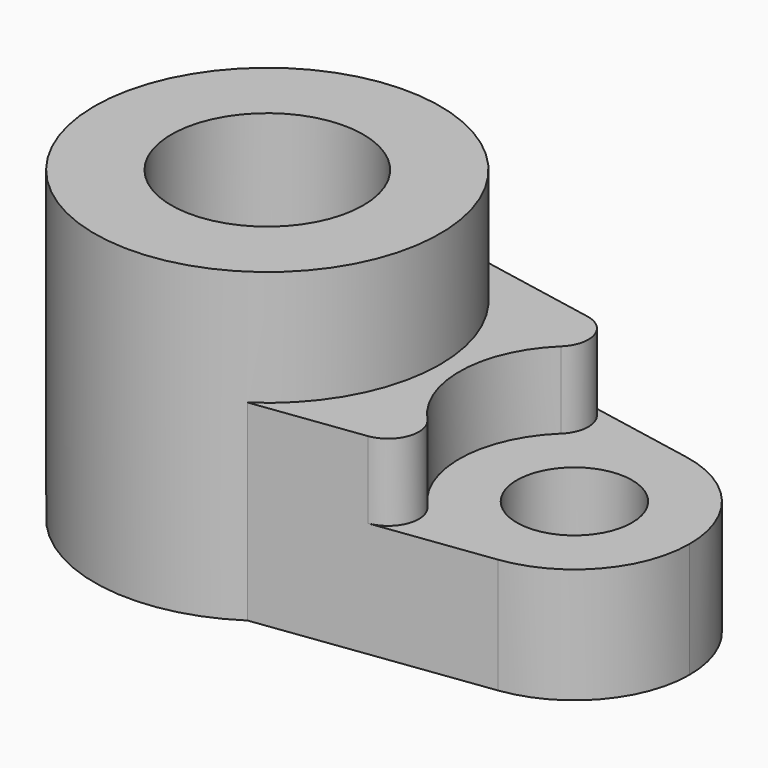
from build123d import *

# Parameters (mm, degrees)
F0_R        = 15.875
F1_DEPTH    = 50.8
F2_DEPTH    = 31.75
F0_R_2      = 9.525
F3_DEPTH    = 19.05
F4_T1_DEPTH = 61.8868884968


# Not quite as in the source:
# - a fillet or chamfer that OpenCascade refuses, or shapes differently, is made with other operations: its cross-section is extruded or revolved along the edge and cut away or added


with BuildPart() as f1:
    # F0 (on Top) → F1 (new body)
    with BuildSketch(Plane.XY):
        with BuildLine():
            ThreePointArc((-25.9736086209, -23.8194207925), (-16.5833436809, -13.5180364382), (-13.1835957324, 0))
            ThreePointArc((-13.1835957324, 0), (-19.7400794655, 18.2130603251), (-36.4007832324, 28.0682110263))
            ThreePointArc((-36.4007832324, 28.0682110263), (-69.7735217146, -5.6297910447), (-25.9736086209, -23.8194207925))
        make_face()
        with Locations((-41.7585957324, 0)):
            Circle(F0_R, mode=Mode.SUBTRACT)
    extrude(amount=F1_DEPTH)

    # F0 (on Top) → F2 (join)
    with BuildSketch(Plane.XY):
        with BuildLine():
            ThreePointArc((-36.4007832324, 28.0682110263), (-19.7400794655, 18.2130603251), (-13.1835957324, 0))
            ThreePointArc((-13.1835957324, 0), (-16.5833436809, -13.5180364382), (-25.9736086209, -23.8194207925))
            Line((-25.9736086209, -23.8194207925), (11.5255643148, -18.8873356739))
            ThreePointArc((11.5255643148, -18.8873356739), (-10.0006293875, 0.5508668403), (12.6132792676, 18.7121406842))
            Line((12.6132792676, 18.7121406842), (-36.4007832324, 28.0682110263))
        make_face()
    extrude(amount=F2_DEPTH)

    # F0 (on Top) → F3 (join)
    with BuildSketch(Plane.XY):
        with BuildLine():
            ThreePointArc((28.0914042676, 0), (23.7204151122, 12.1420402167), (12.6132792676, 18.7121406842))
            ThreePointArc((12.6132792676, 18.7121406842), (-10.0006293875, 0.5508668403), (11.5255643148, -18.8873356739))
            ThreePointArc((11.5255643148, -18.8873356739), (23.3631665352, -12.5614340563), (28.0914042676, 0))
        make_face()
        with Locations((9.0414042676, 0)):
            Circle(F0_R_2, mode=Mode.SUBTRACT)
    extrude(amount=F3_DEPTH)

    # F4: fillet of radius 5.08 on 2 edges, made by hand

    # F4_s2 → F4_t1 (cut)
    with BuildSketch(Plane.XY.offset(19.05)):
        with BuildLine():
            ThreePointArc((-6.7125365301, 22.4011573214), (-2.7943533432, 18.8544597398), (-4.147891099, 13.7457261624))
            ThreePointArc((-4.147891099, 13.7457261624), (3.6293795146, 18.265061951), (12.6132792676, 18.7121406842))
            Line((12.6132792676, 18.7121406842), (-6.7125365301, 22.4011573214))
        make_face()
        with BuildLine():
            ThreePointArc((-7.9811920904, -21.4529651384), (-3.8645283867, -18.1387075787), (-4.9204686565, -12.9602702306))
            ThreePointArc((-4.9204686565, -12.9602702306), (2.5825344428, -17.921648936), (11.5255643148, -18.8873356739))
            Line((11.5255643148, -18.8873356739), (-7.9811920904, -21.4529651384))
        make_face()
    extrude(amount=F4_T1_DEPTH, mode=Mode.SUBTRACT)


solid = f1.part
